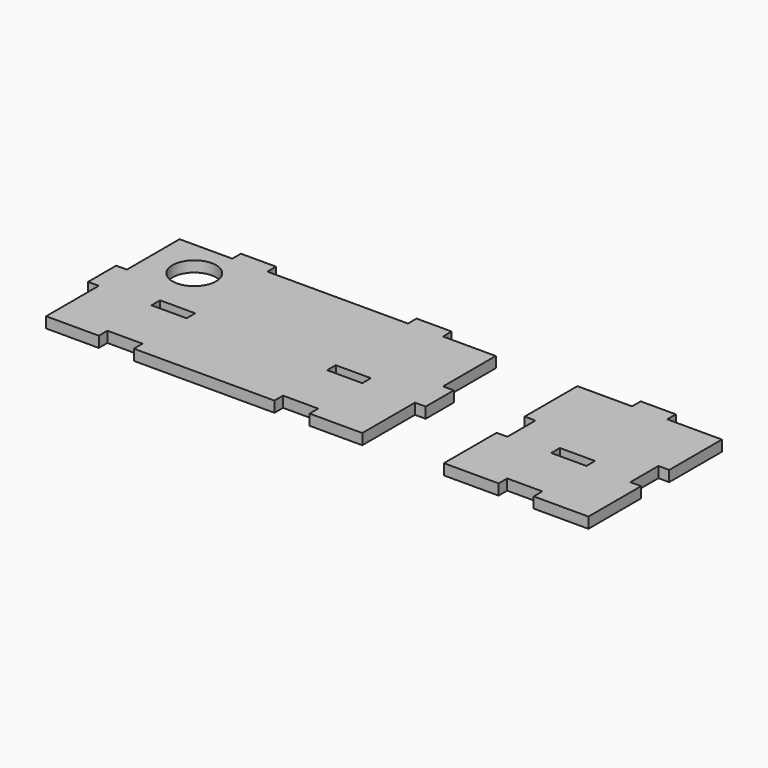
from build123d import *

# Parameters (mm, degrees)
F1_W     = 20
F1_H     = 6.14
F1_R     = 12.4378806179
F1_W_2   = 6.103127097
F1_H_2   = 20
F1_W_3   = 6.102888166
F2_DEPTH = 6.14
F3_DEPTH = 6.14


# Not quite as in the source:
# - a feature names something its author has since deleted; it is built from what else it names


with BuildPart() as f2:
    # F1 (on Top) → F2 (new body)
    with BuildSketch(Plane.XY):
        Polygon((-90.0001194655, -10), (-90.0001194655, -47.5), (-60, -47.5), (-60, -41.36), (-40, -41.36), (-40, -47.5), (40, -47.5), (40, -41.36), (60, -41.36), (60, -47.5), (89.9998805345, -47.5), (89.9998805345, -10), (89.9998805345, 10), (89.9998805345, 47.5), (60, 47.5), (60, 53.64), (40, 53.64), (40, 47.5), (-40, 47.5), (-40, 53.64), (-60, 53.64), (-60, 47.5), (-90.0001194655, 47.5), (-90.0001194655, 10), align=None)
        with Locations((-50, -6.93)):
            Rectangle(F1_W, F1_H, mode=Mode.SUBTRACT)
        with Locations((50, -6.93)):
            Rectangle(F1_W, F1_H, mode=Mode.SUBTRACT)
        with Locations((-64.4147619605, 25.9968824685)):
            Circle(F1_R, mode=Mode.SUBTRACT)
        with Locations((93.051444083, 0)):
            Rectangle(F1_W_2, F1_H_2)
        with Locations((-93.0515635485, 0)):
            Rectangle(F1_W_3, F1_H_2)
    extrude(amount=F2_DEPTH)


with BuildPart() as f3:
    # F1 (on Top) → F3 (new body)
    with BuildSketch(Plane.XY):
        Polygon((218.7568147469, -10), (212.6168147469, -10), (212.6168147469, 10), (218.7568147469, 10), (218.7568147469, 47.5), (187.6168147469, 47.5), (187.6168147469, 53.64), (167.6168147469, 53.64), (167.6168147469, 47.5), (136.4768147469, 47.5), (136.4768147469, 10), (142.6168147469, 10), (142.6168147469, -10), (136.4768147469, -10), (136.4768147469, -47.5), (167.6168147469, -47.5), (167.6168147469, -41.36), (187.6168147469, -41.36), (187.6168147469, -47.5), (218.7568147469, -47.5), align=None)
        with Locations((177.6168147469, -6.93)):
            Rectangle(F1_W, F1_H, mode=Mode.SUBTRACT)
    extrude(amount=F3_DEPTH)


solid = Compound([f2.part, f3.part])
